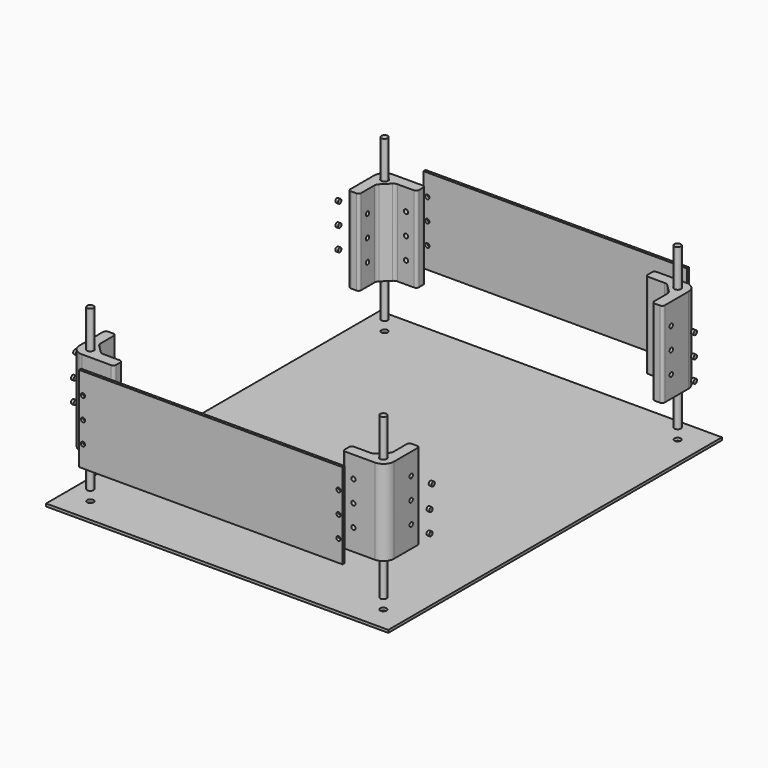
from build123d import *

# Parameters (mm, degrees)
F0_W      = 320
F0_H      = 390
F0_R      = 3
F1_DEPTH  = 2.5
F3_R      = 3
F4_DEPTH  = 150
F8_R      = 3.25
F9_DEPTH  = 80
F10_R     = 2
F11_DEPTH = 377.001
F12_R     = 2
F13_DEPTH = 307.001
F14_R     = 10
F15_R     = 2.5
F16_R     = 5
F20_W     = 246.5
F20_H     = 80
F20_R     = 2
F21_DEPTH = 2.5
F24_R     = 2
F25_DEPTH = 2.5


with BuildPart() as f1:
    # F0 (on Top) → F1 (new body)
    with BuildSketch(Plane.XY):
        Rectangle(F0_W, F0_H)
        with Locations((-137, -172)):
            Circle(F0_R, mode=Mode.SUBTRACT)
        with Locations((137, -172)):
            Circle(F0_R, mode=Mode.SUBTRACT)
        with Locations((-137, 172)):
            Circle(F0_R, mode=Mode.SUBTRACT)
        with Locations((137, 172)):
            Circle(F0_R, mode=Mode.SUBTRACT)
    extrude(amount=F1_DEPTH)


with BuildPart() as f4:
    # F3 (on offset) → F4 (new body)
    with BuildSketch(Plane.XY.offset(12.5)):
        with Locations((-137, -172)):
            Circle(F3_R)
    extrude(amount=F4_DEPTH)


with BuildPart() as f5_1:
    # F5: instance of F4
    add(f4.part.mirror(Plane.YZ))


with BuildPart() as f6_1:
    # F6: instance of F4
    add(f4.part.mirror(Plane.XZ))


with BuildPart() as f6_2:
    # F6: instance of F5_1
    add(f5_1.part.mirror(Plane.XZ))


with BuildPart() as f9:
    # F8 (on offset) → F9 (new body)
    with BuildSketch(Plane.XY.offset(47.5)):
        Polygon((-137, -142), (-147, -142), (-147, -182), (-107, -182), (-107, -172), (-127, -172), (-137, -162), align=None)
        with Locations((-137, -172)):
            Circle(F8_R, mode=Mode.SUBTRACT)
    extrude(amount=F9_DEPTH)

    # F10 (on face) → F11 (cut, through all)
    with BuildSketch(Plane.XZ.offset(182)):
        with Locations((-117, 107.5)):
            Circle(F10_R)
        with Locations((-117, 87.5)):
            Circle(F10_R)
        with Locations((-117, 67.5)):
            Circle(F10_R)
    extrude(amount=-F11_DEPTH, mode=Mode.SUBTRACT)

    # F12 (on face) → F13 (cut, through all)
    with BuildSketch(Plane(origin=(-147, 0, 0), x_dir=(0, -1, 0), z_dir=(-1, 0, 0))):
        with Locations((152, 87.5)):
            Circle(F12_R)
        with Locations((152, 107.5)):
            Circle(F12_R)
        with Locations((152, 67.5)):
            Circle(F12_R)
    extrude(amount=-F13_DEPTH, mode=Mode.SUBTRACT)

    # F14
    f14_edges = [f9.edges().sort_by_distance(p)[0] for p in [
        (-147, -182, 87.5),
    ]]
    fillet(f14_edges, radius=F14_R)

    # F15
    f15_edges = [f9.edges().sort_by_distance(p)[0] for p in [
        (-107, -172, 87.5),
        (-137, -142, 87.5),
        (-147, -142, 87.5),
        (-107, -182, 87.5),
    ]]
    fillet(f15_edges, radius=F15_R)

    # F16
    f16_edges = [f9.edges().sort_by_distance(p)[0] for p in [
        (-137, -162, 87.5),
        (-127, -172, 87.5),
    ]]
    fillet(f16_edges, radius=F16_R)


with BuildPart() as f17_1:
    # F17: instance of F9
    add(f9.part.mirror(Plane.YZ))


with BuildPart() as f18_1:
    # F18: instance of F9
    add(f9.part.mirror(Plane.XZ))


with BuildPart() as f18_2:
    # F18: instance of F17_1
    add(f17_1.part.mirror(Plane.XZ))


with BuildPart() as f21:
    # F20 (on offset) → F21 (new body)
    with BuildSketch(Plane.XZ.offset(200)):
        with Locations((0, 87.5)):
            Rectangle(F20_W, F20_H)
        with Locations((-119.5, 67.5)):
            Circle(F20_R, mode=Mode.SUBTRACT)
        with Locations((119.5, 67.5)):
            Circle(F20_R, mode=Mode.SUBTRACT)
        with Locations((-119.5, 87.5)):
            Circle(F20_R, mode=Mode.SUBTRACT)
        with Locations((-119.5, 107.5)):
            Circle(F20_R, mode=Mode.SUBTRACT)
        with Locations((119.5, 87.5)):
            Circle(F20_R, mode=Mode.SUBTRACT)
        with Locations((119.5, 107.5)):
            Circle(F20_R, mode=Mode.SUBTRACT)
    extrude(amount=F21_DEPTH)


with BuildPart() as f22_1:
    # F22: instance of F21
    add(f21.part.mirror(Plane.XZ))


with BuildPart() as f25:
    # F24 (on offset) → F25 (new body)
    with BuildSketch(Plane.YZ.offset(165)):
        with Locations((-152, 107.5)):
            Circle(F24_R)
    extrude(amount=F25_DEPTH)


with BuildPart() as f25b:
    # F24 (on offset) → F25, piece 2 (new body)
    with BuildSketch(Plane.YZ.offset(165)):
        with Locations((-154.5, 87.5)):
            Circle(F24_R)
    extrude(amount=F25_DEPTH)


with BuildPart() as f25c:
    # F24 (on offset) → F25, piece 3 (new body)
    with BuildSketch(Plane.YZ.offset(165)):
        with Locations((-154.5, 67.5)):
            Circle(F24_R)
    extrude(amount=F25_DEPTH)


with BuildPart() as f25d:
    # F24 (on offset) → F25, piece 4 (new body)
    with BuildSketch(Plane.YZ.offset(165)):
        with Locations((154.5, 107.5)):
            Circle(F24_R)
    extrude(amount=F25_DEPTH)


with BuildPart() as f25e:
    # F24 (on offset) → F25, piece 5 (new body)
    with BuildSketch(Plane.YZ.offset(165)):
        with Locations((154.5, 87.5)):
            Circle(F24_R)
    extrude(amount=F25_DEPTH)


with BuildPart() as f25f:
    # F24 (on offset) → F25, piece 6 (new body)
    with BuildSketch(Plane.YZ.offset(165)):
        with Locations((154.5, 67.5)):
            Circle(F24_R)
    extrude(amount=F25_DEPTH)


with BuildPart() as f26_1:
    # F26: instance of F25
    add(f25.part.mirror(Plane.YZ))


with BuildPart() as f26_2:
    # F26: instance of F25b
    add(f25b.part.mirror(Plane.YZ))


with BuildPart() as f26_3:
    # F26: instance of F25c
    add(f25c.part.mirror(Plane.YZ))


with BuildPart() as f26_4:
    # F26: instance of F25d
    add(f25d.part.mirror(Plane.YZ))


with BuildPart() as f26_5:
    # F26: instance of F25e
    add(f25e.part.mirror(Plane.YZ))


with BuildPart() as f26_6:
    # F26: instance of F25f
    add(f25f.part.mirror(Plane.YZ))


solid = Compound([f1.part, f4.part, f5_1.part, f6_1.part, f6_2.part, f9.part, f17_1.part, f18_1.part, f18_2.part, f21.part, f22_1.part, f25.part, f25b.part, f25c.part, f25d.part, f25e.part, f25f.part, f26_1.part, f26_2.part, f26_3.part, f26_4.part, f26_5.part, f26_6.part])
